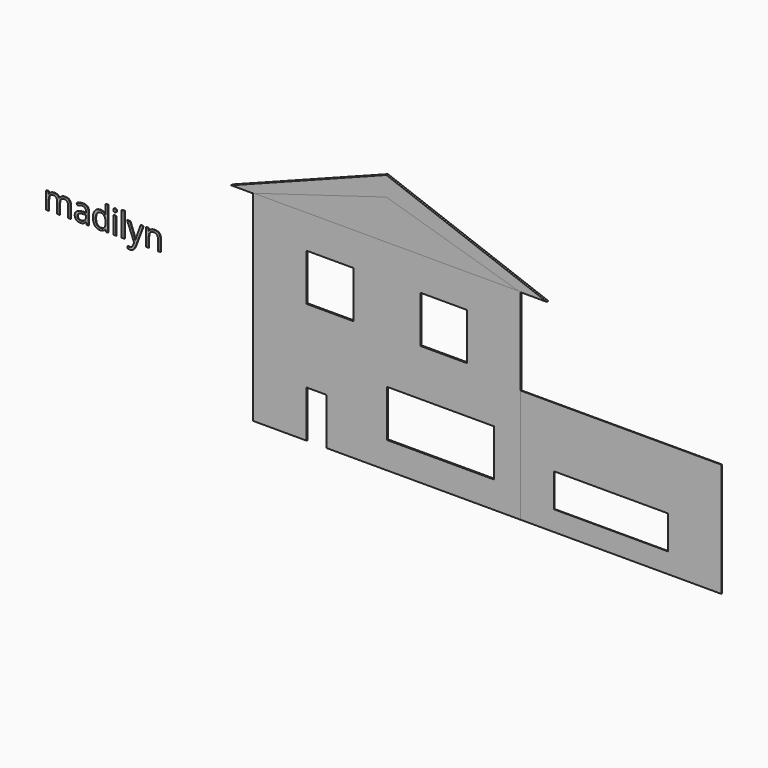
from build123d import *

# Parameters (mm, degrees)
F0_TEXT_SIZE = 1465.3209182951
F0_W         = 4876.8
F0_H         = 2133.6
F0_W_2       = 2133.6
F1_DEPTH     = 30.48
F0_W_3       = 9144
F0_H_2       = 3962.4
F0_W_4       = 5181.6
F0_H_3       = 1524
F0_H_4       = 1219.2
F2_DEPTH     = 30.48
F3_DEPTH     = 30.48
F4_DEPTH     = 30.48
F5_DEPTH     = 30.48


# Not quite as in the source:
# - Text() gives the source's letters only with a copy of the font that has no kerning and outlines rounded to 1/6400 em; it was checked with that copy


with BuildPart() as f1:
    # F0 (on Front) → F1 (new body)
    with BuildSketch(Plane.XZ):
        with Locations((-15675.0755310059, -3768.5985565186)):
            Text('madilyn', F0_TEXT_SIZE, font='Open Sans', text_align=(TextAlign.LEFT, TextAlign.BOTTOM))
        Polygon((0, 914.4), (0, 0), (6096, 0), (0, 1828.8), align=None)
        Polygon((-6096, 0), (0, 0), (0, 914.4), (0, 1828.8), align=None)
        Polygon((0, 1828.8), (6096, 0), (7314.2495653036, 0), (0, 2713.1133079529), (-7072.3352432251, 0), (-6096, 0), align=None)
        Polygon((6096, 0), (0, 0), (-6096, 0), (-6096, -9144), (-3657.6, -9144), (-3657.6, -7010.4), (-2743.2, -7010.4), (-2743.2, -9144), (6096, -9144), (6096, -5181.6), (6096, -3962.4), align=None)
        with Locations((2438.4, -6858)):
            Rectangle(F0_W, F0_H, mode=Mode.SUBTRACT)
        with Locations((-2590.8, -2590.8)):
            Rectangle(F0_W_2, F0_H, mode=Mode.SUBTRACT)
        with Locations((2590.8, -2590.8)):
            Rectangle(F0_W_2, F0_H, mode=Mode.SUBTRACT)
    extrude(amount=-F1_DEPTH)

    # F0 (on Front) → F2 (join)
    with BuildSketch(Plane.XZ):
        Polygon((0, 1828.8), (6096, 0), (7314.2495653036, 0), (0, 2713.1133079529), (-7072.3352432251, 0), (-6096, 0), align=None)
        with Locations((10668, -7162.8)):
            Rectangle(F0_W_3, F0_H_2)
        with Locations((10210.8, -7467.6)):
            Rectangle(F0_W_4, F0_H_3, mode=Mode.SUBTRACT)
        with Locations((10668, -4572)):
            Rectangle(F0_W_3, F0_H_4)
    extrude(amount=F2_DEPTH)

    # F3 (add): a face of the model
    f3_faces = [f1.faces().sort_by_distance(p)[0] for p in [
        (-3090.0682413769, -30.48, 1054.6274712563),
    ]]
    extrude(f3_faces, amount=F3_DEPTH)

    # F0 (on Front) → F4 (join)
    with BuildSketch(Plane.XZ):
        Polygon((-6096, 0), (0, 0), (0, 914.4), (0, 1828.8), align=None)
        Polygon((0, 914.4), (0, 0), (6096, 0), (0, 1828.8), align=None)
    extrude(amount=F4_DEPTH)


with BuildPart() as f5:
    # F0 (on Front) → F5 (new body)
    with BuildSketch(Plane.XZ):
        Polygon((6096, 0), (0, 0), (-6096, 0), (-6096, -9144), (-3657.6, -9144), (-3657.6, -7010.4), (-2743.2, -7010.4), (-2743.2, -9144), (6096, -9144), (6096, -5181.6), (6096, -3962.4), align=None)
        with Locations((2438.4, -6858)):
            Rectangle(F0_W, F0_H, mode=Mode.SUBTRACT)
        with Locations((-2590.8, -2590.8)):
            Rectangle(F0_W_2, F0_H, mode=Mode.SUBTRACT)
        with Locations((2590.8, -2590.8)):
            Rectangle(F0_W_2, F0_H, mode=Mode.SUBTRACT)
    extrude(amount=F5_DEPTH)


solid = Compound([f1.part, f5.part])
